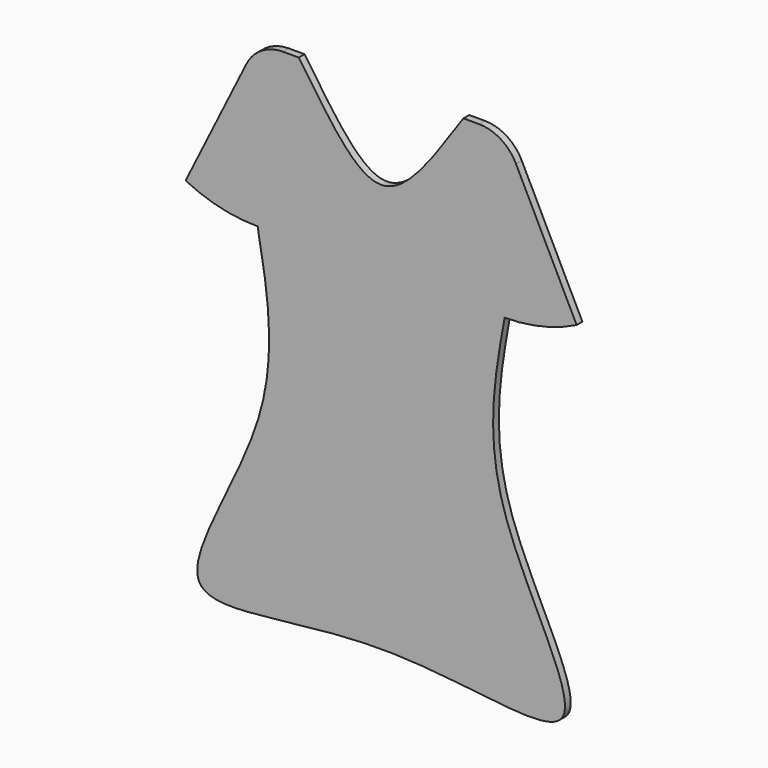
from build123d import *

# Parameters (mm, degrees)
F1_DEPTH = 8.89


with BuildPart() as f1:
    # F0 (on Front) → F1 (new body)
    with BuildSketch(Plane.XZ):
        with BuildLine():
            ThreePointArc((-120.8973585091, 0), (-147.6699706341, -7.6274712346), (-166.4029241427, -28.2194))
            Line((-166.4029241427, -28.2194), (-241.3, -179.1557702113))
            ThreePointArc((-241.3, -179.1557702113), (-198.0554813672, -194.7192261209), (-152.4, -200))
            add(Edge.make_bspline(
                [(-152.4, -200), (-140.4639950109, -266.9888747602), (-114.6109354207, -399.4931685645), (-304.3956902598, -671.6410884783), (-109.977203101, -609.6), (0, -609.6)],
                knots=[0, 0, 0, 0, 0.3300414219, 0.6598179581, 1, 1, 1, 1], degree=3))
            add(Edge.make_bspline(
                [(152.4, -200), (140.4639950109, -266.9888747602), (114.6109354207, -399.4931685645), (304.3956902598, -671.6410884783), (109.977203101, -609.6), (0, -609.6)],
                knots=[0, 0, 0, 0, 0.3300414219, 0.6598179581, 1, 1, 1, 1], degree=3))
            ThreePointArc((152.4, -200), (198.0554813672, -194.7192261209), (241.3, -179.1557702113))
            Line((241.3, -179.1557702113), (166.4029241427, -28.2194))
            ThreePointArc((166.4029241427, -28.2194), (147.6699706341, -7.6274712346), (120.8973585091, 0))
            Line((120.8973585091, 0), (101.6, 0))
            add(Edge.make_bspline(
                [(101.6, 0), (65.2, -52.6007674634), (0, -157.8023023903), (-65.2, -52.6007674634), (-101.6, 0)],
                knots=[0, 0, 0, 0, 0.5, 1, 1, 1, 1], degree=3))
            Line((-101.6, 0), (-120.8973585091, 0))
        make_face()
    extrude(amount=F1_DEPTH)


solid = f1.part
